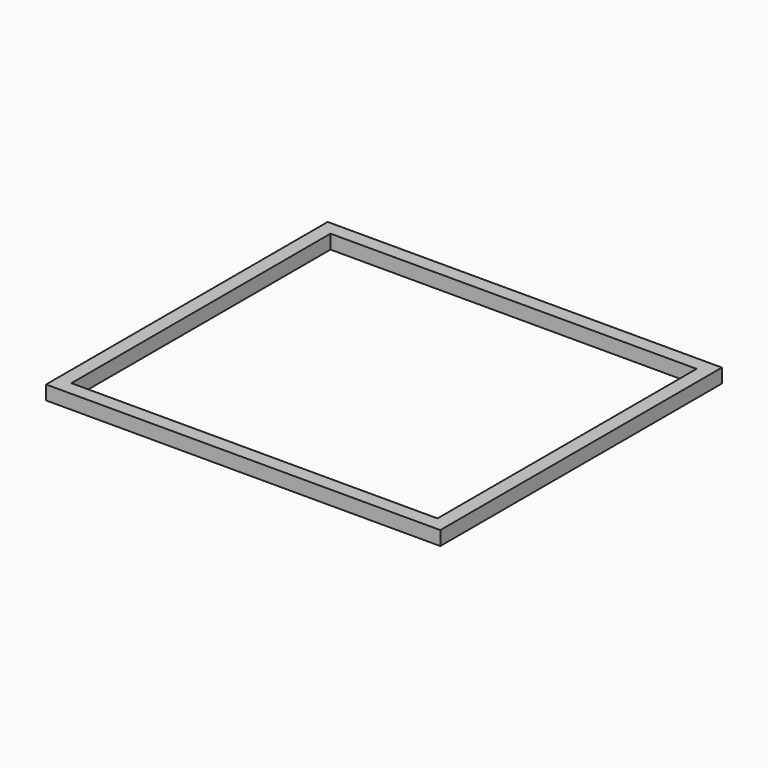
from build123d import *

# Parameters (mm, degrees)
F1_W = 25.4
F1_H = 25.4


with BuildPart() as f2:
    # F2: sweep along a path in F0
    with BuildLine(Plane.XY) as f2_path:
        Line((-330.2, 292.1), (-330.2, -292.1))
        Line((-330.2, -292.1), (330.2, -292.1))
        Line((330.2, -292.1), (330.2, 292.1))
        Line((330.2, 292.1), (-330.2, 292.1))
    # F1 (on Front) → F2 (sweep)
    with BuildSketch(Plane.XZ):
        with Locations((-342.9, 0)):
            Rectangle(F1_W, F1_H)
    sweep(path=f2_path.line, transition=Transition.RIGHT)


solid = f2.part
